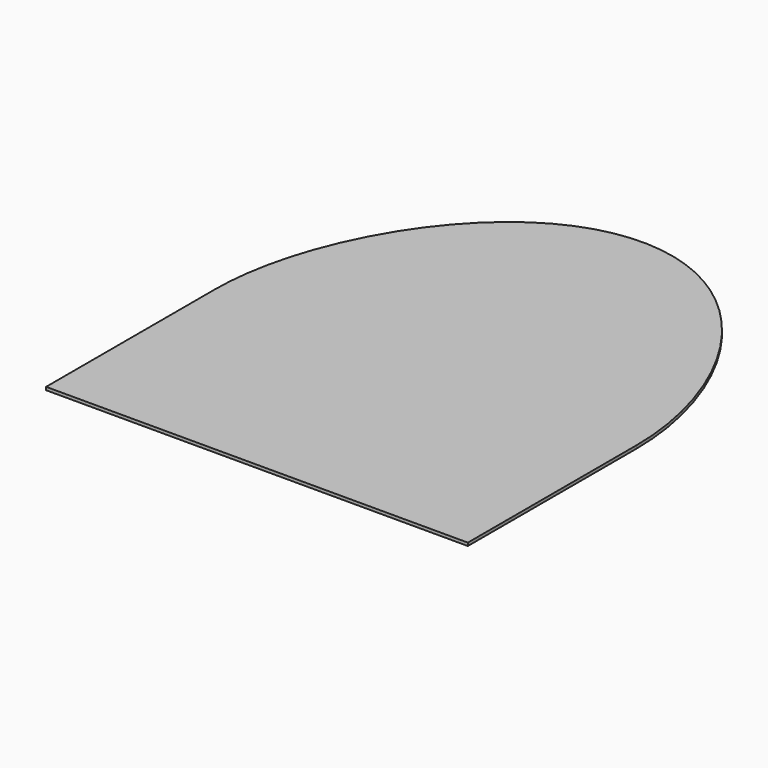
from build123d import *

# Parameters (mm, degrees)
F1_DEPTH = 0.5


# Not quite as in the source:
# - ends of sketch curves that miss each other by under 0.0002 mm in the source are joined


with BuildPart() as f1:
    # F0 (on Top) → F1 (new body)
    with BuildSketch(Plane.XY):
        with BuildLine():
            Line((-35, 2.1762e-06), (-35, -35))
            Line((-35, -35), (-27, -35))
            Line((-27, -35), (-27, -22.2710574513))
            ThreePointArc((-27, -22.2710574513), (-32.9393385518, -11.8321585422), (-35, 2.1762e-06))
        make_face()
        with BuildLine():
            Line((-27, -22.2710574513), (-27, -35))
            Line((-27, -35), (0, -35))
            ThreePointArc((0, -35), (-14.9250291324, -31.658229663), (-27, -22.2710574513))
        make_face()
        with BuildLine():
            ThreePointArc((27, -22.2710574513), (14.9250291324, -31.658229663), (0, -35))
            Line((0, -35), (27, -35))
            Line((27, -35), (27, -22.2710574513))
        make_face()
        with BuildLine():
            Line((27, -22.2710574513), (27, -35))
            Line((27, -35), (35, -35))
            Line((35, -35), (35, 0))
            ThreePointArc((35, 0), (32.939338184, -11.8321595662), (27, -22.2710574513))
        make_face()
        with BuildLine():
            add(Edge.make_bspline(
                [(0, 45), (-20.1986748725, 45), (-35, 20.0504870868), (-35, 2.1762e-06)],
                knots=[0, 0, 0, 0, 57.0087695372, 57.0087695372, 57.0087695372, 57.0087695372], degree=3))
            ThreePointArc((-35, 2.1762e-06), (-28.4666369261, 20.3629708568), (-11.3056830814, 33.1237306181))
            add(Edge.make_bspline(
                [(0, 37), (-0.2833414452, 37.0069688983), (-1.1232932293, 37.0068386903), (-2.7957299856, 36.8864035146), (-4.9942322029, 36.3521195303), (-7.6997383876, 35.2871018647), (-9.7958540485, 34.148638444), (-11.0540635502, 33.3003360386), (-11.3056830814, 33.1237306181)],
                knots=[0, 0, 0, 0, 0.8506820357, 2.5185967411, 5.0181648841, 7.6012051941, 11.2266191262, 12.1476935207, 12.1476935207, 12.1476935207, 12.1476935207], degree=3))
            add(Edge.make_bspline(
                [(0, 37), (0.2833414452, 37.0069688983), (1.1232932293, 37.0068386903), (2.7957299856, 36.8864035146), (4.9942322029, 36.3521195303), (7.6997383876, 35.2871018647), (9.7958540485, 34.148638444), (11.0540635502, 33.3003360386), (11.3056830814, 33.1237306181)],
                knots=[0, 0, 0, 0, 0.8506820357, 2.5185967411, 5.0181648841, 7.6012051941, 11.2266191262, 12.1476935207, 12.1476935207, 12.1476935207, 12.1476935207], degree=3))
            ThreePointArc((11.3056830814, 33.1237306181), (28.4666375592, 20.3629699719), (35, 0))
            add(Edge.make_bspline(
                [(0, 45), (20.1986748725, 45), (35, 20.0504870868), (35, 0)],
                knots=[0, 0, 0, 0, 57.0087695372, 57.0087695372, 57.0087695372, 57.0087695372], degree=3))
        make_face()
        with BuildLine():
            Line((27, 2.1762e-06), (27, -22.2710574513))
            ThreePointArc((27, -22.2710574513), (32.939338184, -11.8321595662), (35, 0))
            ThreePointArc((35, 0), (28.4666375592, 20.3629699719), (11.3056830814, 33.1237306181))
            add(Edge.make_bspline(
                [(11.3056830814, 33.1237306181), (12.4097508436, 32.3488132243), (15.1414824386, 30.0752135158), (18.8876274503, 25.5283101279), (22.422035633, 19.604279738), (25.0662594291, 13.1120426553), (26.6478130576, 7.1844788974), (27.0173066601, 2.7756083867), (27.018694794, 0.6711028041), (27, 2.1762e-06)],
                knots=[12.1476935207, 12.1476935207, 12.1476935207, 12.1476935207, 16.189226149, 22.7543847852, 29.7183326598, 36.8091409701, 43.7289829573, 48.0262708445, 50.0404462243, 50.0404462243, 50.0404462243, 50.0404462243], degree=3))
        make_face()
        with BuildLine():
            ThreePointArc((-11.3056830814, 33.1237306181), (-28.4666369261, 20.3629708568), (-35, 2.1762e-06))
            ThreePointArc((-35, 2.1762e-06), (-32.9393385518, -11.8321585422), (-27, -22.2710574513))
            Line((-27, -22.2710574513), (-27, 2.1762e-06))
            add(Edge.make_bspline(
                [(-11.3056830814, 33.1237306181), (-12.4097508436, 32.3488132243), (-15.1414824386, 30.0752135158), (-18.8876274503, 25.5283101279), (-22.422035633, 19.604279738), (-25.0662594291, 13.1120426553), (-26.6478130576, 7.1844788974), (-27.0173066601, 2.7756083867), (-27.018694794, 0.6711028041), (-27, 2.1762e-06)],
                knots=[12.1476935207, 12.1476935207, 12.1476935207, 12.1476935207, 16.189226149, 22.7543847852, 29.7183326598, 36.8091409701, 43.7289829573, 48.0262708445, 50.0404462243, 50.0404462243, 50.0404462243, 50.0404462243], degree=3))
        make_face()
        with BuildLine():
            ThreePointArc((-27, -22.2710574513), (-14.9250291324, -31.658229663), (0, -35))
            ThreePointArc((0, -35), (14.9250291324, -31.658229663), (27, -22.2710574513))
            Line((27, -22.2710574513), (27, 2.1762e-06))
            add(Edge.make_bspline(
                [(11.3056830814, 33.1237306181), (12.4097508436, 32.3488132243), (15.1414824386, 30.0752135158), (18.8876274503, 25.5283101279), (22.422035633, 19.604279738), (25.0662594291, 13.1120426553), (26.6478130576, 7.1844788974), (27.0173066601, 2.7756083867), (27.018694794, 0.6711028041), (27, 2.1762e-06)],
                knots=[12.1476935207, 12.1476935207, 12.1476935207, 12.1476935207, 16.189226149, 22.7543847852, 29.7183326598, 36.8091409701, 43.7289829573, 48.0262708445, 50.0404462243, 50.0404462243, 50.0404462243, 50.0404462243], degree=3))
            ThreePointArc((11.3056830814, 33.1237306181), (0, 35), (-11.3056830814, 33.1237306181))
            add(Edge.make_bspline(
                [(-11.3056830814, 33.1237306181), (-12.4097508436, 32.3488132243), (-15.1414824386, 30.0752135158), (-18.8876274503, 25.5283101279), (-22.422035633, 19.604279738), (-25.0662594291, 13.1120426553), (-26.6478130576, 7.1844788974), (-27.0173066601, 2.7756083867), (-27.018694794, 0.6711028041), (-27, 2.1762e-06)],
                knots=[12.1476935207, 12.1476935207, 12.1476935207, 12.1476935207, 16.189226149, 22.7543847852, 29.7183326598, 36.8091409701, 43.7289829573, 48.0262708445, 50.0404462243, 50.0404462243, 50.0404462243, 50.0404462243], degree=3))
            Line((-27, 2.1762e-06), (-27, -22.2710574513))
        make_face()
        with BuildLine():
            add(Edge.make_bspline(
                [(0, 37), (-0.2833414452, 37.0069688983), (-1.1232932293, 37.0068386903), (-2.7957299856, 36.8864035146), (-4.9942322029, 36.3521195303), (-7.6997383876, 35.2871018647), (-9.7958540485, 34.148638444), (-11.0540635502, 33.3003360386), (-11.3056830814, 33.1237306181)],
                knots=[0, 0, 0, 0, 0.8506820357, 2.5185967411, 5.0181648841, 7.6012051941, 11.2266191262, 12.1476935207, 12.1476935207, 12.1476935207, 12.1476935207], degree=3))
            ThreePointArc((-11.3056830814, 33.1237306181), (0, 35), (11.3056830814, 33.1237306181))
            add(Edge.make_bspline(
                [(0, 37), (0.2833414452, 37.0069688983), (1.1232932293, 37.0068386903), (2.7957299856, 36.8864035146), (4.9942322029, 36.3521195303), (7.6997383876, 35.2871018647), (9.7958540485, 34.148638444), (11.0540635502, 33.3003360386), (11.3056830814, 33.1237306181)],
                knots=[0, 0, 0, 0, 0.8506820357, 2.5185967411, 5.0181648841, 7.6012051941, 11.2266191262, 12.1476935207, 12.1476935207, 12.1476935207, 12.1476935207], degree=3))
        make_face()
    extrude(amount=F1_DEPTH)


solid = f1.part
